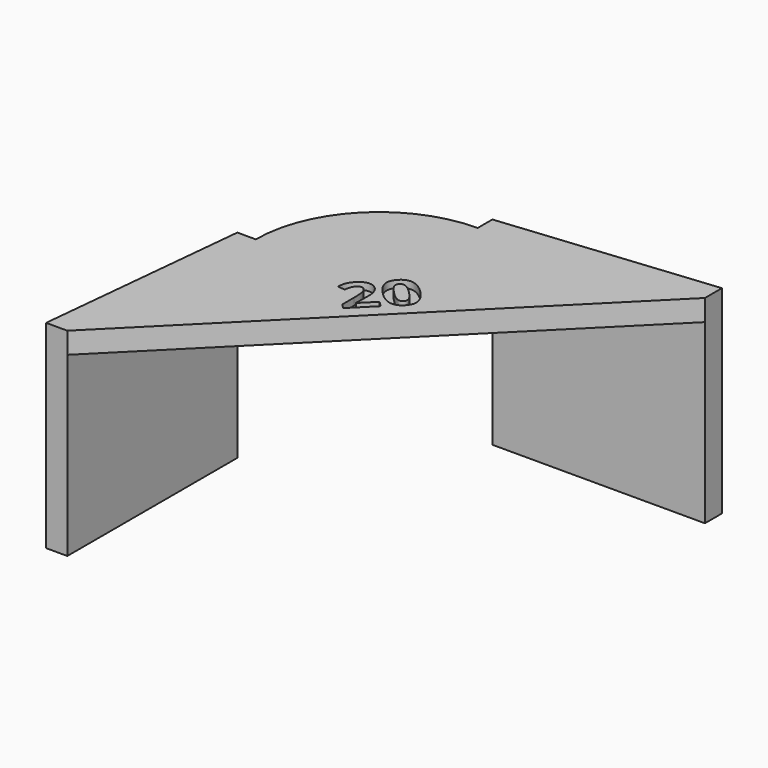
from build123d import *

# Parameters (mm, degrees)
F1_DEPTH     = 3
F2_SIZE      = 2.6
F3_DEPTH     = 3
F4_DEPTH     = 25
F5_TEXT_SIZE = 8.3333333333
F6_DEPTH     = 1


# Not quite as in the source:
# - Text() gives the source's letters only with a copy of the font that has no kerning and outlines rounded to 1/6400 em; it was checked with that copy


with BuildPart() as f1:
    # F0 (on Top) → F1 (new body)
    with BuildSketch(Plane.XY):
        with BuildLine():
            Line((0, 0), (0, 20))
            ThreePointArc((0, 20), (-14.1421356237, 14.1421356237), (-20, 0))
            Line((-20, 0), (0, 0))
        make_face()
    extrude(amount=F1_DEPTH)

    # F2
    f2_edges = [f1.edges().sort_by_distance(p)[0] for p in [
        (-14.142136, 14.142136, 3),
    ]]
    chamfer(f2_edges, length=F2_SIZE)

    # F0 (on Top) → F3 (join, through all)
    with BuildSketch(Plane.XY):
        Polygon((30, 20), (0, 20), (0, 0), (-20, 0), (-20, -30), align=None)
        Polygon((30, 23), (0, 20), (30, 20), align=None)
        Polygon((-20, -30), (-20, 0), (-23, -30), align=None)
    extrude(amount=F3_DEPTH)

    # F0 (on Top) → F4 (join)
    with BuildSketch(Plane.XY):
        Polygon((30, 23), (0, 20), (30, 20), align=None)
        Polygon((-20, -30), (-20, 0), (-23, -30), align=None)
    extrude(amount=-F4_DEPTH)

    # F5 (on face) → F6 (cut)
    with BuildSketch(Plane.XY.offset(3)):
        with Locations(Location((0.1363390995, -7.0352337758), (0, 0, 45))):
            Text('20', F5_TEXT_SIZE, font='Open Sans', font_style=FontStyle.BOLD, text_align=(TextAlign.LEFT, TextAlign.BOTTOM))
    extrude(amount=-F6_DEPTH, mode=Mode.SUBTRACT)


solid = f1.part
